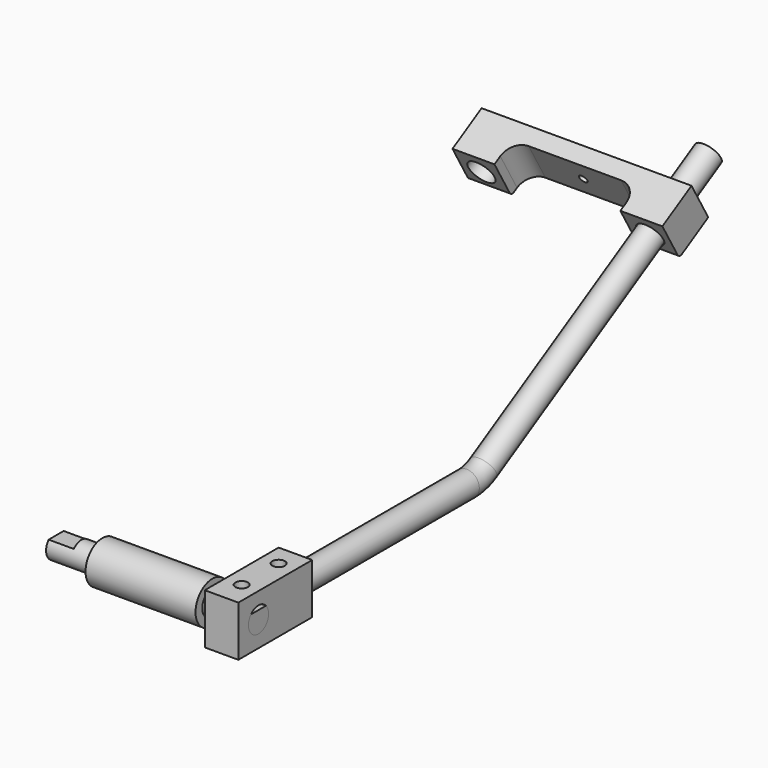
from build123d import *

# Parameters (mm, degrees)
F0_R      = 5
F1_DEPTH  = 24.1
F2_R      = 5
F2_R_2    = 3
F3_DEPTH  = 11
F4_R      = 5
F4_R_2    = 3
F5_DEPTH  = 11
F7_DEPTH  = 6
F9_DEPTH  = 6
F10_W     = 22
F10_H     = 12
F11_DEPTH = 8
F12_R     = 3
F13_DEPTH = 48.201
F14_R     = 3
F15_DEPTH = 9
F16_R     = 1.5
F17_REACH = 16.2436406871
F18_R     = 1.5
F19_REACH = 16.2436406871
F20_R     = 3
F25_DEPTH = 4
F27_W     = 50
F27_H     = 10
F27_R     = 3.15
F27_R_2   = 1
F28_DEPTH = 10
F29_W     = 30
F29_H     = 6
F30_DEPTH = 45.5881685741
F31_R     = 4
F32_R     = 1


with BuildPart() as f1:
    # F0 (on Right) → F1 (new body, symmetric)
    with BuildSketch(Plane.YZ):
        Circle(F0_R)
    extrude(amount=F1_DEPTH, both=True)

    # F2 (on face) → F3 (cut)
    with BuildSketch(Plane.YZ.offset(24.1)):
        Circle(F2_R)
        Circle(F2_R_2, mode=Mode.SUBTRACT)
    extrude(amount=-F3_DEPTH, mode=Mode.SUBTRACT)

    # F4 (on face) → F5 (cut)
    with BuildSketch(Plane(origin=(-24.1, 0, 0), x_dir=(0, -1, 0), z_dir=(-1, 0, 0))):
        Circle(F4_R)
        Circle(F4_R_2, mode=Mode.SUBTRACT)
    extrude(amount=-F5_DEPTH, mode=Mode.SUBTRACT)

    # F6 (on face) → F7 (cut)
    with BuildSketch(Plane.YZ.offset(24.1)):
        with BuildLine():
            ThreePointArc((2.2360679775, 2), (0, 3), (-2.2360679775, 2))
            Line((-2.2360679775, 2), (2.2360679775, 2))
        make_face()
    extrude(amount=-F7_DEPTH, mode=Mode.SUBTRACT)

    # F8 (on face) → F9 (cut)
    with BuildSketch(Plane(origin=(-24.1, 0, 0), x_dir=(0, -1, 0), z_dir=(-1, 0, 0))):
        with BuildLine():
            Line((-2.2360679775, 2), (2.2360679775, 2))
            ThreePointArc((2.2360679775, 2), (0, 3), (-2.2360679775, 2))
        make_face()
    extrude(amount=-F9_DEPTH, mode=Mode.SUBTRACT)


with BuildPart() as f11:
    # F10 (on face) → F11 (new body)
    with BuildSketch(Plane.YZ.offset(24.1)):
        with Locations((5, 0)):
            Rectangle(F10_W, F10_H)
    extrude(amount=-F11_DEPTH)

    # F12 (on face) → F13 (cut, through all)
    with BuildSketch(Plane.YZ.offset(24.1)):
        Circle(F12_R)
    extrude(amount=-F13_DEPTH, mode=Mode.SUBTRACT)

    # F14 (on face) → F15 (cut)
    with BuildSketch(Plane(origin=(0, 16, 0), x_dir=(-1, 0, 0), z_dir=(0, 1, 0))):
        with Locations((-20.1, 0)):
            Circle(F14_R)
    extrude(amount=-F15_DEPTH, mode=Mode.SUBTRACT)

    f17_end = f11.faces().sort_by_distance((20.1, -3, 0))[0]
    # F16 (on face) → F17 (cut, up to a face of the model that its end follows)
    with BuildSketch(Plane.XY.offset(6)):
        with Locations((20.1, 0)):
            Circle(F16_R)
    f17_long = extrude(amount=-F17_REACH, mode=Mode.PRIVATE)
    add(split(f17_long, bisect_by=f17_end, keep=Keep.ALL, mode=Mode.PRIVATE).solids().sort_by_distance((20.1, 0, 6))[0], mode=Mode.SUBTRACT)

    f19_end = f11.faces().sort_by_distance((23.1, 11.5, 0))[0]
    # F18 (on face) → F19 (cut, up to a face of the model that its end follows)
    with BuildSketch(Plane.XY.offset(6)):
        with Locations((20.1, 11)):
            Circle(F18_R)
    f19_long = extrude(amount=-F19_REACH, mode=Mode.PRIVATE)
    add(split(f19_long, bisect_by=f19_end, keep=Keep.ALL, mode=Mode.PRIVATE).solids().sort_by_distance((20.1, 11, 6))[0], mode=Mode.SUBTRACT)


with BuildPart() as f22:
    # F22: sweep along a path in F21
    with BuildLine(Plane.YZ) as f22_path:
        Line((7, 0), (67, 0))
        ThreePointArc((67, 0), (69.588190451, 0.3407417371), (72, 1.3397459622))
        Line((72, 1.3397459622), (138.9615242271, 40))
    # F20 (on face) → F22 (sweep)
    with BuildSketch(Plane(origin=(0, 7, 0), x_dir=(-1, 0, 0), z_dir=(0, 1, 0))):
        with Locations((-20.1, 0)):
            Circle(F20_R)
    sweep(path=f22_path.line)

    # F24 (on offset) → F25 (cut)
    with BuildSketch(Plane.XZ.offset(-9)):
        with BuildLine():
            Line((17.8639320225, 2), (22.3360679775, 2))
            ThreePointArc((22.3360679775, 2), (20.1, 3), (17.8639320225, 2))
        make_face()
    extrude(amount=-F25_DEPTH, mode=Mode.SUBTRACT)


with BuildPart() as f28:
    # F27 (on offset) → F28 (new body)
    with BuildSketch(Plane(origin=(0, 104.2211431703, 60.1721050646), x_dir=(-1, 0, 0), z_dir=(0, 0.8660254038, 0.5))):
        with Locations((0, -34.8397459622)):
            Rectangle(F27_W, F27_H)
        with Locations((-20.1, -34.8397459622)):
            Circle(F27_R, mode=Mode.SUBTRACT)
        with Locations((0, -34.8397459622)):
            Circle(F27_R_2, mode=Mode.SUBTRACT)
        with Locations((20.1, -34.8397459622)):
            Circle(F27_R, mode=Mode.SUBTRACT)
    extrude(amount=F28_DEPTH)

    # F29 (on face) → F30 (cut, through all)
    with BuildSketch(Plane(origin=(0, 14.9198729811, -25.8419780457), x_dir=(1, 0, 0), z_dir=(0, -0.5, 0.8660254038))):
        with Locations((0, 123.3442101292)):
            Rectangle(F29_W, F29_H)
    extrude(amount=-F30_DEPTH, mode=Mode.SUBTRACT)

    # F31
    f31_edges = [f28.edges().sort_by_distance(p)[0] for p in [
        (-15, 126.837169, 33),
        (15, 126.837169, 33),
    ]]
    fillet(f31_edges, radius=F31_R)

    # F32
    f32_edges = [f28.edges().sort_by_distance(p)[0] for p in [
        (20, 124.141016, 25.669873),
        (-20, 124.141016, 25.669873),
    ]]
    fillet(f32_edges, radius=F32_R)


solid = Compound([f1.part, f11.part, f22.part, f28.part])
